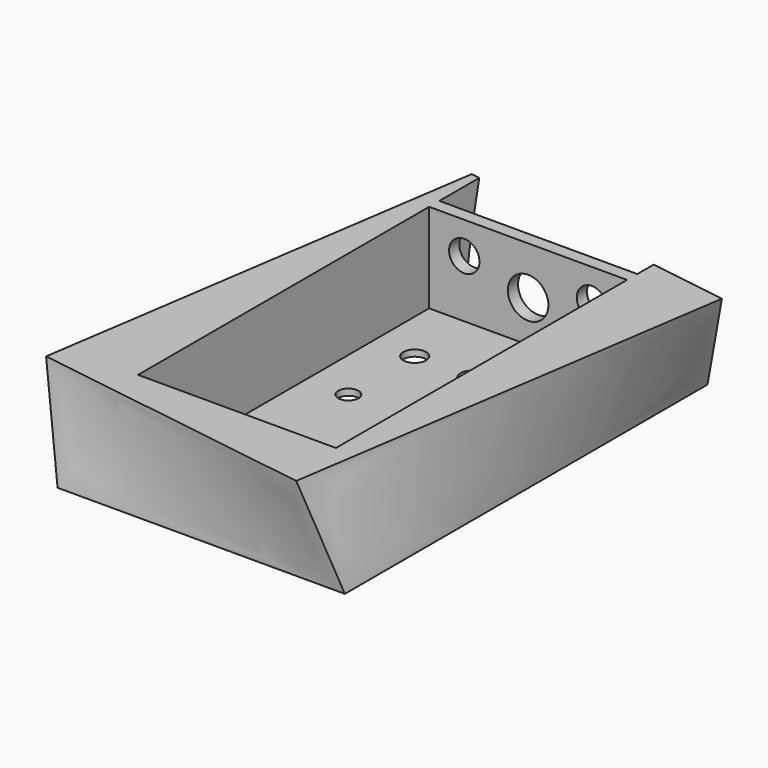
from build123d import *

# Parameters (mm, degrees)
F0_W            = 70
F0_H            = 122
F1_DEPTH        = 30
F2_W            = 90
F2_H            = 142
F5_W            = 62
F5_H            = 114
F6_DEPTH        = 28
F7_R            = 3.571875
F7_R_2          = 3.175
F7_R_3          = 6.35
F8_DEPTH        = 25
F9_R            = 6.35
F9_R_2          = 4.7625
F10_DEPTH       = 25
F12_TEXT_SIZE   = 4.6780206125
F12_TEXT_SIZE_2 = 4.7208352247
F12_TEXT_SIZE_3 = 4.7372316802
F13_DEPTH       = 1
F15_W           = 62
F15_H           = 28
F16_DEPTH       = 25


# Not quite as in the source:
# - Text() gives the source's letters only with a copy of the font that has no kerning and outlines rounded to 1/6400 em; it was checked with that copy


with BuildPart() as f1:
    # F0 (on Top) → F1 (new body)
    with BuildSketch(Plane.XY):
        Rectangle(F0_W, F0_H)
    extrude(amount=F1_DEPTH)

    # F2 (on face) → F4 section 0
    with BuildSketch(Plane(origin=(0, 0, 0), x_dir=(1, 0, 0), z_dir=(0, 0, -1))):
        Rectangle(F2_W, F2_H)
    # F3 (on face) → F4 section 1
    with BuildSketch(Plane.XY.offset(30)):
        Polygon((55.3245018899, 63.7334266519), (-33.6869258127, 77.0362736536), (-54.6758621931, -63.4039789438), (34.3355655095, -76.7068259455), align=None)
    loft()

    # F5 (on face) → F6 (cut)
    with BuildSketch(Plane.XY.offset(30)):
        Rectangle(F5_W, F5_H)
    extrude(amount=-F6_DEPTH, mode=Mode.SUBTRACT)

    # F7 (on face) → F8 (cut)
    with BuildSketch(Plane.XY.offset(2)):
        with Locations((-17.9119046929, 35)):
            Circle(F7_R)
        with Locations((0, 35)):
            Circle(F7_R)
        with Locations((17.9119046929, 35)):
            Circle(F7_R)
        with Locations((17.9119046929, 9)):
            Circle(F7_R_2)
        with Locations((0, -38)):
            Circle(F7_R_3)
        with Locations((-17.9119046929, 9)):
            Circle(F7_R_2)
    extrude(amount=-F8_DEPTH, mode=Mode.SUBTRACT)

    # F9 (on face) → F10 (cut)
    with BuildSketch(Plane.XZ.offset(-57)):
        with Locations((0, 15)):
            Circle(F9_R)
        with Locations((20, 20)):
            Circle(F9_R_2)
        with Locations((-20, 20)):
            Circle(F9_R_2)
    extrude(amount=-F10_DEPTH, mode=Mode.SUBTRACT)

    # F12 (on face) → F13 (cut)
    with BuildSketch(Plane(origin=(0, 0, 0), x_dir=(1, 0, 0), z_dir=(0, 0, -1))):
        with Locations(Location((29.4715252517, -21.631825159), (0, 0, 180))):
            Text('VOLUME', F12_TEXT_SIZE, font='Open Sans', font_style=FontStyle.BOLD, text_align=(TextAlign.LEFT, TextAlign.BOTTOM))
        with Locations(Location((6.3406735292, -21.6009986382), (0, 0, 180))):
            Text('TONE', F12_TEXT_SIZE_2, font='Open Sans', font_style=FontStyle.BOLD, text_align=(TextAlign.LEFT, TextAlign.BOTTOM))
        with Locations(Location((-12.8297237973, -21.5891931902), (0, 0, 180))):
            Text('GAIN', F12_TEXT_SIZE_3, font='Open Sans', font_style=FontStyle.BOLD, text_align=(TextAlign.LEFT, TextAlign.BOTTOM))
    extrude(amount=-F13_DEPTH, mode=Mode.SUBTRACT)

    # F15 (on offset) → F16 (cut)
    with BuildSketch(Plane.XZ.offset(-61)):
        with Locations((0, 16)):
            Rectangle(F15_W, F15_H)
    extrude(amount=-F16_DEPTH, mode=Mode.SUBTRACT)


solid = f1.part
